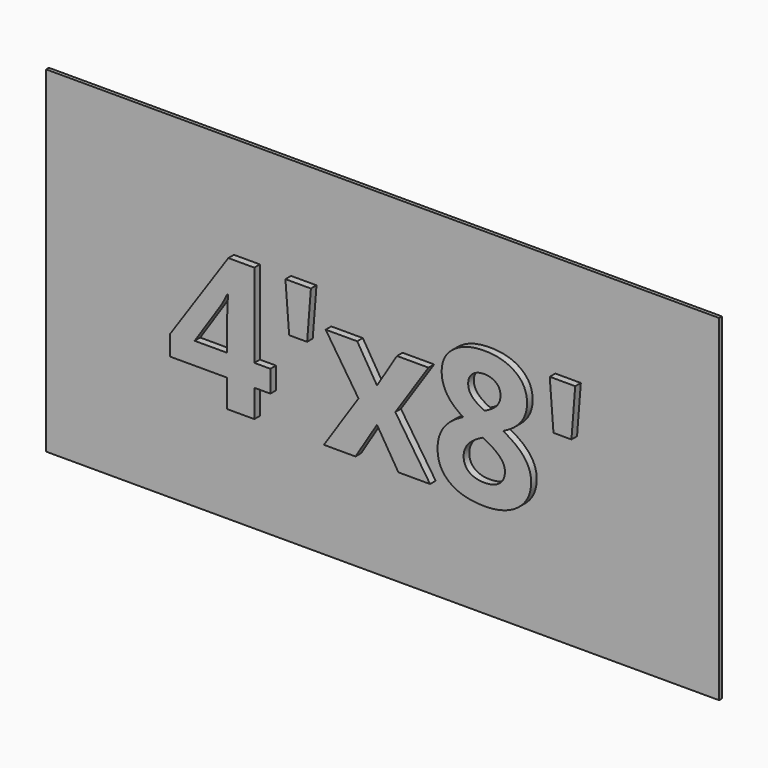
from build123d import *

# Parameters (mm, degrees)
F0_W         = 2438.4
F0_H         = 1219.2
F1_DEPTH     = 12.7
F2_TEXT_SIZE = 676.7693588676
F3_DEPTH     = 25.4
F4_TEXT_SIZE = 676.7693588676
F5_DEPTH     = 25.4


# Not quite as in the source:
# - Text() gives the source's letters only with a copy of the font that has no kerning and outlines rounded to 1/6400 em; it was checked with that copy


with BuildPart() as f1:
    # F0 (on Front) → F1 (new body)
    with BuildSketch(Plane.XZ):
        with Locations((1219.2, 609.6)):
            Rectangle(F0_W, F0_H)
    extrude(amount=F1_DEPTH)

    # F2 (on face) → F3 (join)
    with BuildSketch(Plane.XZ.offset(12.7)):
        with Locations((457.2, 365.9630308077)):
            Text("4'x8'", F2_TEXT_SIZE, font='Open Sans', font_style=FontStyle.BOLD, text_align=(TextAlign.LEFT, TextAlign.BOTTOM))
    extrude(amount=F3_DEPTH)

    # F4 (on face) → F5 (join)
    with BuildSketch(Plane(origin=(0, 0, 0), x_dir=(-1, 0, 0), z_dir=(0, 1, 0))):
        with Locations((-1981.2, 365.9630308077)):
            Text("4'x8'", F4_TEXT_SIZE, font='Open Sans', font_style=FontStyle.BOLD, text_align=(TextAlign.LEFT, TextAlign.BOTTOM))
    extrude(amount=F5_DEPTH)


solid = f1.part
